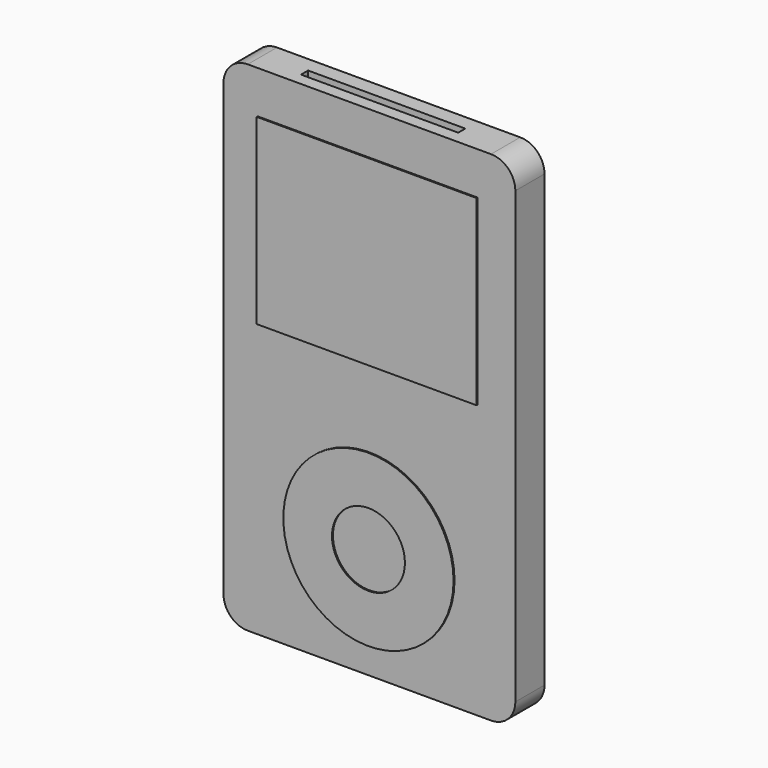
from build123d import *

# Parameters (mm, degrees)
F0_W        = 60.96
F0_H        = 104.14
F1_DEPTH    = 7.62
F2_W        = 45.9153815961
F2_H        = 38.1
F2_R        = 17.78
F2_R_2      = 7.62
F3_DEPTH    = 0.254
F4_W        = 13.0856782198
F4_H        = 1.975195948
F5_DEPTH    = 2.54
F6_R        = 2.2527466913
F7_DEPTH    = 2.54
F8_T1_DEPTH = 33.02
F9_W        = 32.8376358375
F9_H        = 1.8517468125
F10_DEPTH   = 2.54


# Not quite as in the source:
# - a fillet or chamfer that OpenCascade refuses, or shapes differently, is made with other operations: its cross-section is extruded or revolved along the edge and cut away or added


with BuildPart() as f1:
    # F0 (on Front) → F1 (new body)
    with BuildSketch(Plane.XZ):
        with Locations((-22.7986111199, 3.2297596335)):
            Rectangle(F0_W, F0_H)
    extrude(amount=F1_DEPTH)

    # F2 (on face) → F3 (join)
    with BuildSketch(Plane.XZ.offset(7.62)):
        with Locations((-23.1955593918, 27.3597596335)):
            Rectangle(F2_W, F2_H)
        with Locations((-22.7986111199, -25.5444776267)):
            Circle(F2_R)
        with Locations((-22.7986111199, -25.5444776267)):
            Circle(F2_R_2, mode=Mode.SUBTRACT)
    extrude(amount=F3_DEPTH)

    # F4 (on face) → F5 (cut)
    with BuildSketch(Plane(origin=(0, 0, -48.8402403665), x_dir=(1, 0, 0), z_dir=(0, 0, -1))):
        with Locations((-44.3373024464, 3.3156641293)):
            Rectangle(F4_W, F4_H)
    extrude(amount=-F5_DEPTH, mode=Mode.SUBTRACT)

    # F6 (on face) → F7 (cut)
    with BuildSketch(Plane(origin=(0, 0, -48.8402403665), x_dir=(1, 0, 0), z_dir=(0, 0, -1))):
        with Locations((-1.6869211104, 4.2321491055)):
            Circle(F6_R)
    extrude(amount=-F7_DEPTH, mode=Mode.SUBTRACT)

    # F8: fillet of radius 5.08 on 4 edges, made by hand

    # F8_s2 → F8_t1 (cut)
    with BuildSketch(Plane.XZ.offset(-12.7)):
        with BuildLine():
            ThreePointArc((2.6013888801, 55.2997596335), (6.1934913285, 53.811862082), (7.6813888801, 50.2197596335))
            Line((7.6813888801, 50.2197596335), (7.6813888801, 55.2997596335))
            Line((7.6813888801, 55.2997596335), (2.6013888801, 55.2997596335))
        make_face()
        with BuildLine():
            ThreePointArc((-48.1986111199, 55.2997596335), (-51.7907135683, 53.811862082), (-53.2786111199, 50.2197596335))
            Line((-53.2786111199, 50.2197596335), (-53.2786111199, 55.2997596335))
            Line((-53.2786111199, 55.2997596335), (-48.1986111199, 55.2997596335))
        make_face()
        with BuildLine():
            ThreePointArc((7.6813888801, -43.7602403665), (6.1934913285, -47.3523428149), (2.6013888801, -48.8402403665))
            Line((2.6013888801, -48.8402403665), (7.6813888801, -48.8402403665))
            Line((7.6813888801, -48.8402403665), (7.6813888801, -43.7602403665))
        make_face()
        with BuildLine():
            ThreePointArc((-53.2786111199, -43.7602403665), (-51.7907135683, -47.3523428149), (-48.1986111199, -48.8402403665))
            Line((-48.1986111199, -48.8402403665), (-53.2786111199, -48.8402403665))
            Line((-53.2786111199, -48.8402403665), (-53.2786111199, -43.7602403665))
        make_face()
    extrude(amount=F8_T1_DEPTH, mode=Mode.SUBTRACT)

    # F9 (on face) → F10 (cut)
    with BuildSketch(Plane.XY.offset(55.2997596335)):
        with Locations((-22.7386062033, -4.1089197621)):
            Rectangle(F9_W, F9_H)
    extrude(amount=-F10_DEPTH, mode=Mode.SUBTRACT)


solid = f1.part
